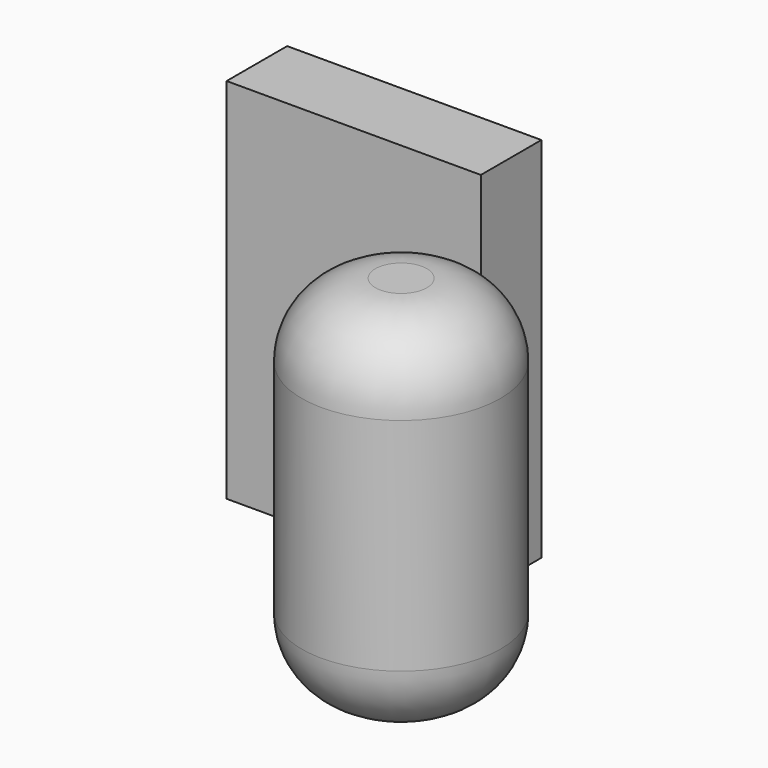
from build123d import *

# Parameters (mm, degrees)
F1_W     = 17.5571227446
F1_H     = 5.2252039313
F2_DEPTH = 25.4
F0_R     = 6.8614235902
F3_DEPTH = 25.4
F6_R     = 5.08


# Not quite as in the source:
# - the program builds the solid bodies; features that only make, move or delete a surface that nothing else refers to are left out


with BuildPart() as f2:
    # F1 (on Top) → F2 (new body)
    with BuildSketch(Plane.XY):
        with Locations((-12.9580865614, 14.7183928639)):
            Rectangle(F1_W, F1_H)
    extrude(amount=F2_DEPTH)


with BuildPart() as f3:
    # F0 (on Top) → F3 (new body)
    with BuildSketch(Plane.XY):
        Circle(F0_R)
    extrude(amount=F3_DEPTH)

    # F6
    f6_edges = [f3.edges().sort_by_distance(p)[0] for p in [
        (6.861424, 0, 12.7),
        (-6.861424, 0, 0),
        (-6.861424, 0, 25.4),
    ]]
    fillet(f6_edges, radius=F6_R)


solid = Compound([f2.part, f3.part])
